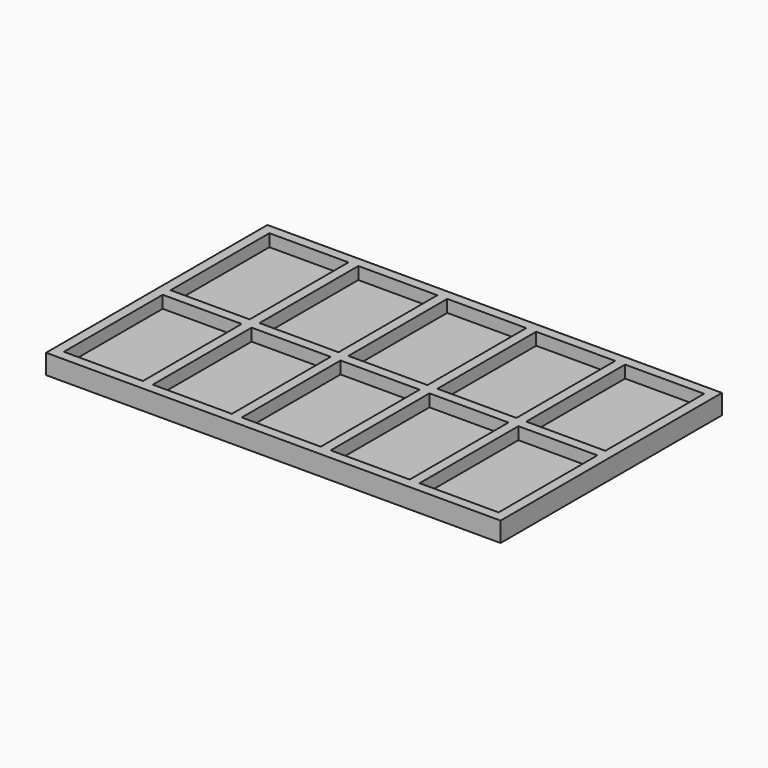
from build123d import *

# Parameters (mm, degrees)
F0_W      = 92
F0_H      = 56
F1_DEPTH  = 1.5
F2_W      = 2
F2_H      = 56
F3_DEPTH  = 4
F5_W      = 92
F5_H      = 2
F6_DEPTH  = 4
F8_W      = 2
F8_H      = 56
F9_DEPTH  = 4
F11_W     = 2
F11_H     = 56
F12_DEPTH = 4
F14_W     = 92
F14_H     = 2
F15_DEPTH = 4


# Not quite as in the source:
# - a feature names something its author has since deleted; it is built from what else it names


with BuildPart() as f1:
    # F0 (on Top) → F1 (new body)
    with BuildSketch(Plane.XY):
        Rectangle(F0_W, F0_H)
    extrude(amount=F1_DEPTH)

    # F4: F3 across plane


with BuildPart() as f3:
    # F2 (on Top) → F3 (new body)
    with BuildSketch(Plane.XY):
        with Locations((45, 0)):
            Rectangle(F2_W, F2_H)
    extrude(amount=F3_DEPTH)


with BuildPart() as f1_1:
    add(f1.part)
    add(f3.part.mirror(Plane.YZ))


    add(f3.part)  # F6 merges F3
    # F5 (on Top) → F6 (join)
    with BuildSketch(Plane.XY):
        with Locations((0, -27)):
            Rectangle(F5_W, F5_H)
    extrude(amount=F6_DEPTH)

    # F7: F1 across plane


with BuildPart() as f1_2:
    add(f1_1.part)
    add(f1_1.part.mirror(Plane.XZ))

    # F8 (on Top) → F9 (join)
    with BuildSketch(Plane.XY):
        with Locations((27, 0)):
            Rectangle(F8_W, F8_H)
    extrude(amount=F9_DEPTH)

    # F10: F1 across plane


with BuildPart() as f1_3:
    add(f1_2.part)
    add(f1_2.part.mirror(Plane.YZ))

    # F11 (on Top) → F12 (join)
    with BuildSketch(Plane.XY):
        with Locations((9, 0)):
            Rectangle(F11_W, F11_H)
    extrude(amount=F12_DEPTH)

    # F13: F1 across plane


with BuildPart() as f1_4:
    add(f1_3.part)
    add(f1_3.part.mirror(Plane.YZ))

    # F14 (on Top) → F15 (join)
    with BuildSketch(Plane.XY):
        Rectangle(F14_W, F14_H)
    extrude(amount=F15_DEPTH)


solid = f1_4.part
